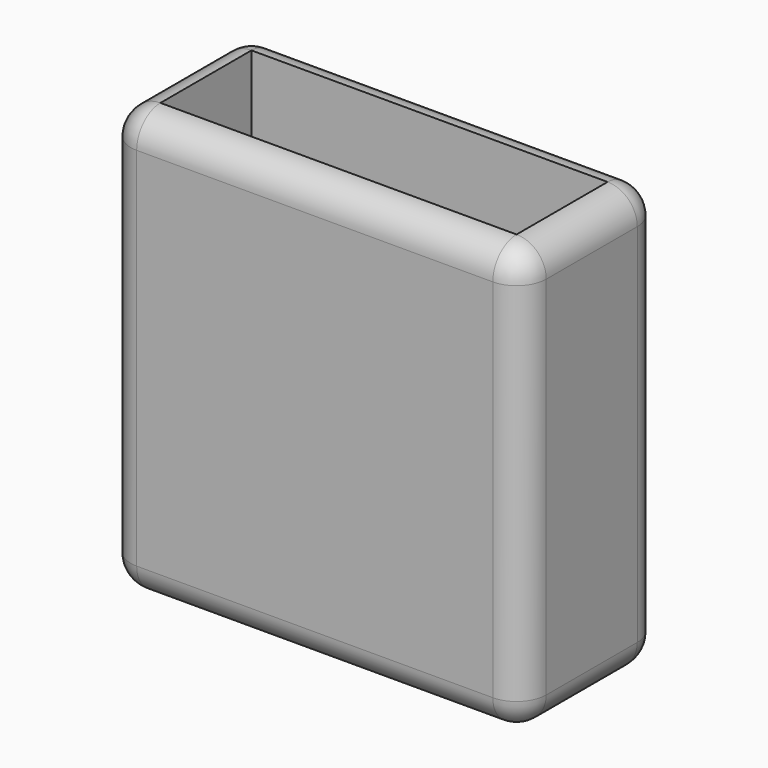
from build123d import *

# Parameters (mm, degrees)
F0_W     = 42
F0_H     = 17.5
F0_W_2   = 36
F0_H_2   = 11.5
F1_DEPTH = 40
F2_DEPTH = 3
F3_R     = 3
F4_R     = 2.99999


# Not quite as in the source:
# - a fillet or chamfer is up to 0.001 mm smaller than in the source, because OpenCascade refuses the exact size


with BuildPart() as f1:
    # F0 (on Top) → F1 (new body)
    with BuildSketch(Plane.XY):
        with Locations((12.1359585822, -3.1205574796)):
            Rectangle(F0_W, F0_H)
        with Locations((12.1359585822, -3.1205574796)):
            Rectangle(F0_W_2, F0_H_2, mode=Mode.SUBTRACT)
    extrude(amount=F1_DEPTH)

    # F0 (on Top) → F2 (join)
    with BuildSketch(Plane.XY):
        with Locations((12.1359585822, -3.1205574796)):
            Rectangle(F0_W, F0_H)
        with Locations((12.1359585822, -3.1205574796)):
            Rectangle(F0_W_2, F0_H_2, mode=Mode.SUBTRACT)
        with Locations((12.1359585822, -3.1205574796)):
            Rectangle(F0_W_2, F0_H_2)
    extrude(amount=-F2_DEPTH)

    # F3
    f3_edges = [f1.edges().sort_by_distance(p)[0] for p in [
        (33.135959, -11.870557, 18.5),
        (12.135959, -11.870557, -3),
        (33.135959, -3.120557, -3),
        (33.135959, 5.629443, 18.5),
        (12.135959, 5.629443, -3),
        (-8.864041, 5.629443, 18.5),
        (-8.864041, -3.120557, -3),
        (-8.864041, -11.870557, 18.5),
    ]]
    fillet(f3_edges, radius=F3_R)

    # F4 (radius 3 in the source; OpenCascade refuses exactly that, so slightly less here)
    f4_edges = [f1.edges().sort_by_distance(p)[0] for p in [
        (12.135959, 5.629443, 40),
        (-8.864041, -3.120557, 40),
        (12.135959, -11.870557, 40),
        (33.135959, -3.120557, 40),
    ]]
    fillet(f4_edges, radius=F4_R)


solid = f1.part
